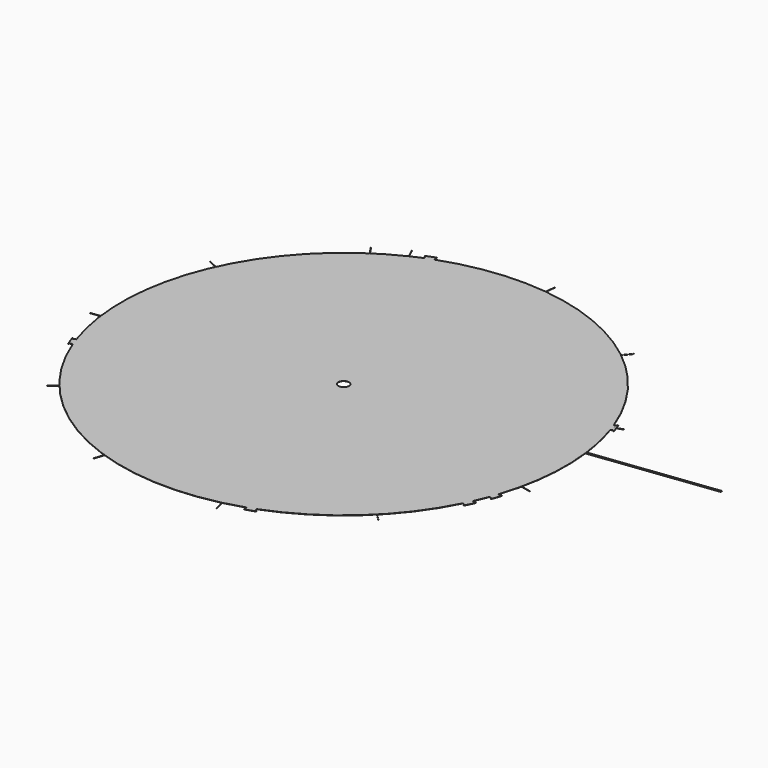
from build123d import *

# Parameters (mm, degrees)
F1_DEPTH = 25.4
F2_R     = 647.7634116636
F3_DEPTH = 25.401
F4_DEPTH = 25.4
F5_COUNT = 12
F5_ANGLE = 352
F6_DEPTH = 25.4


# Not quite as in the source:
# - a feature names something its author has since deleted; it is built from what else it names


with BuildPart() as f1:
    # F0 (on Top) → F1 (new body)
    with BuildSketch(Plane.XY):
        with BuildLine():
            ThreePointArc((26581.7811350736, -5958.878580492), (27076.0679663897, -2997.6433626178), (27241.5, 0))
            ThreePointArc((27241.5, 0), (27192.4503772419, 1634.0026717349), (27045.4781413478, 3262.1211436546))
            Line((27045.4781413478, 3262.1211436546), (27038.1674766005, 3322.1712414177))
            ThreePointArc((27038.1674766005, 3322.1712414177), (27037.0795725779, 3330.3759714052), (27036.1058084748, 3338.5950293075))
            Line((27036.1058084748, 3338.5950293075), (27020.3930406274, 3463.767050483))
            ThreePointArc((27020.3930406274, 3463.767050483), (26566.042215611, 6028.6584949201), (25868.7948916266, 8538.4291942343))
            ThreePointArc((25868.7948916266, 8538.4291942343), (25785.7588811485, 8786.0093997942), (25700.3534370753, 9032.7822656928))
            ThreePointArc((25700.3534370753, 9032.7822656928), (25616.6335659034, 9267.545899548), (25530.7692626016, 9501.5337240783))
            ThreePointArc((25530.7692626016, 9501.5337240783), (22069.8067791267, 15969.4380296244), (17008.4904706443, 21279.3461873245))
            ThreePointArc((17008.4904706443, 21279.3461873245), (10484.2276785736, 25143.1957442532), (3147.6824871739, 27059.0357775354))
            ThreePointArc((3147.6824871739, 27059.0357775354), (-3180.6458046722, 27055.1809181757), (-9337.3289859723, 25591.2799534865))
            ThreePointArc((-9337.3289859723, 25591.2799534865), (-9812.9319890637, 25412.7072156433), (-10285.1222620802, 25225.2964760389))
            ThreePointArc((-10285.1222620802, 25225.2964760389), (-10981.6553363056, 24929.9532355075), (-11669.7181895388, 24615.3813626104))
            Line((-11669.7181895388, 24615.3813626104), (-11694.1794219061, 24603.7698310293))
            ThreePointArc((-11694.1794219061, 24603.7698310293), (-13359.8135246141, 23740.5708616608), (-14962.0879305602, 22764.7808469176))
            ThreePointArc((-14962.0879305602, 22764.7808469176), (-20665.0527895609, 17749.7863495497), (-24761.9849194556, 11355.325847313))
            ThreePointArc((-24761.9849194556, 11355.325847313), (-26932.6996094687, 4090.1117339412), (-27016.7600861348, -3491.9903634219))
            ThreePointArc((-27016.7600861348, -3491.9903634219), (-26537.9717507115, -6151.0468709349), (-25798.1369417149, -8749.5972813909))
            ThreePointArc((-25798.1369417149, -8749.5972813909), (-25630.4432474664, -9229.2849770936), (-25453.8311641421, -9705.7612435783))
            ThreePointArc((-25453.8311641421, -9705.7612435783), (-23563.6007310159, -13669.5297226812), (-21061.0389912676, -17278.0774063061))
            ThreePointArc((-21061.0389912676, -17278.0774063061), (-15482.6864890933, -22413.9630884511), (-8704.7879531066, -25813.2909359006))
            ThreePointArc((-8704.7879531066, -25813.2909359006), (-1252.4719720801, -27212.6925571351), (6296.8812891127, -26503.7470611388))
            ThreePointArc((6296.8812891127, -26503.7470611388), (7526.087542552, -26181.2400117306), (8738.915501307, -25801.7572678881))
            ThreePointArc((8738.915501307, -25801.7572678881), (9218.6681255216, -25634.2637936316), (9695.2130745943, -25457.8507672627))
            ThreePointArc((9695.2130745943, -25457.8507672627), (14879.2922381078, -22818.9829909877), (19384.9043310167, -19139.6135365198))
            ThreePointArc((19384.9043310167, -19139.6135365198), (22160.1999290659, -15843.7641156964), (24381.1200669519, -12151.555724716))
            ThreePointArc((24381.1200669519, -12151.555724716), (24603.4987154748, -11694.7498138109), (24817.3195457392, -11233.8761260159))
            ThreePointArc((24817.3195457392, -11233.8761260159), (25183.6009790471, -10386.797580493), (25520.9793035129, -9527.7981527564))
            ThreePointArc((25520.9793035129, -9527.7981527564), (25693.4049537871, -9052.5280519151), (25856.9806436038, -8574.1398546034))
            ThreePointArc((25856.9806436038, -8574.1398546034), (26251.9681567532, -7275.5405398372), (26581.7811350736, -5958.878580492))
        make_face()
        with BuildLine():
            Line((26219.4698221007, -8697.857158849), (25856.9806436038, -8574.1398546033))
            ThreePointArc((25856.9806436038, -8574.1398546034), (25693.4049537871, -9052.5280519151), (25520.9793035129, -9527.7981527564))
            Line((25520.9793035128, -9527.7981527565), (25892.889499643, -9654.7308437612))
            Line((25892.889499643, -9654.7308437612), (26219.4698221007, -8697.857158849))
        make_face()
        Polygon((26260.4914258481, -8577.6646964148), (26219.4698221007, -8697.857158849), (25892.889499643, -9654.7308437612), (25850.2700590491, -9779.6049355713), (25922.390865835, -9804.2022830051), (26127.4988845718, -9203.2399708342), (26332.6069033086, -8602.2776586632), align=None)
        with BuildLine():
            Line((25167.4813878364, -11405.5197307459), (24817.3195457391, -11233.876126016))
            ThreePointArc((24817.3195457392, -11233.8761260159), (24603.4987154748, -11694.7498138109), (24381.1200669519, -12151.555724716))
            Line((24381.1200669517, -12151.5557247163), (24720.2908078015, -12317.8116714798))
            Line((24720.2908078015, -12317.8116714798), (25167.4813878364, -11405.5197307459))
        make_face()
        with BuildLine():
            ThreePointArc((25700.3534370753, 9032.7822656928), (25785.7588811485, 8786.0093997942), (25868.7948916266, 8538.4291942343))
            Line((25868.7948916267, 8538.4291942341), (26198.5379395342, 8651.0553115066))
            Line((26198.5379395342, 8651.0553115066), (26028.7355470907, 9148.1971803935))
            Line((26028.7355470907, 9148.1971803935), (25700.3534370753, 9032.7822656928))
        make_face()
        Polygon((25223.3802103407, -11291.4832381542), (25167.4813878364, -11405.5197307459), (24720.2908078015, -12317.8116714798), (24664.3847231965, -12431.8629791328), (24732.8138808522, -12465.3874575742), (25012.307993374, -11895.2049946155), (25291.8021058958, -11325.0225316568), align=None)
        with BuildLine():
            ThreePointArc((25530.7692626016, 9501.5337240783), (25616.6335659034, 9267.545899548), (25700.3534370753, 9032.7822656928))
            Line((25700.3534370753, 9032.7822656928), (26028.7355470907, 9148.1971803935))
            Line((26028.7355470907, 9148.1971803935), (25868.6350307326, 9616.9342150529))
            Line((25868.6350307326, 9616.9342150529), (25530.7692626015, 9501.5337240786))
        make_face()
        Polygon((26028.7355470907, 9148.1971803935), (26198.5379395342, 8651.0553115066), (26238.0846514917, 8535.2717468115), (26310.1891088702, 8559.9169795832), (26104.9422822996, 9160.8318988377), (26100.62746037, 9173.4646927998), align=None)
        Polygon((25868.6350307326, 9616.9342150529), (26028.7355470907, 9148.1971803935), (26100.62746037, 9173.4646927998), (25899.695455729, 9761.7468180923), (25827.5856654185, 9737.1171989038), align=None)
        with BuildLine():
            Line((9817.5292529223, -25823.5618318769), (9695.2130745944, -25457.8507672626))
            ThreePointArc((9695.2130745943, -25457.8507672627), (9218.6681255216, -25634.2637936316), (8738.915501307, -25801.7572678881))
            Line((8738.9155013075, -25801.7572678879), (8853.993553604, -26145.8271823865))
            Line((8853.993553604, -26145.8271823865), (9817.5292529223, -25823.5618318769))
        make_face()
        Polygon((9937.9712153371, -25783.2786630632), (9817.5292529223, -25823.5618318769), (8853.993553604, -26145.8271823865), (8733.5359439607, -26186.1155845918), (8757.7214924774, -26258.3755286491), (9359.9313045514, -26056.9596845806), (9962.1411166253, -25855.5438405121), align=None)
        with BuildLine():
            ThreePointArc((-10285.1222620802, 25225.2964760389), (-9812.9319890637, 25412.7072156433), (-9337.3289859723, 25591.2799534865))
            Line((-9337.3289859723, 25591.2799534865), (-9480.2259121424, 25961.3424129862))
            Line((-9480.2259121424, 25961.3424129862), (-10428.0191882503, 25595.3589355386))
            Line((-10428.0191882503, 25595.3589355386), (-10285.1222620802, 25225.2964760389))
        make_face()
        Polygon((-10428.0191882503, 25595.3589355386), (-9480.2259121424, 25961.3424129862), (-9361.7363610477, 26007.0962910142), (-9389.2005134374, 26078.1748433752), (-9981.5713110049, 25849.4351699704), (-10573.9421085723, 25620.6954965657), (-10546.4933477638, 25549.6110008576), align=None)
        with BuildLine():
            Line((-25797.5388182234, -9838.4814533939), (-25453.8311641418, -9705.7612435791))
            ThreePointArc((-25453.8311641421, -9705.7612435783), (-25630.4432474664, -9229.2849770936), (-25798.1369417149, -8749.5972813909))
            Line((-25798.1369417149, -8749.5972813911), (-26163.522295671, -8890.688177286))
            Line((-26163.522295671, -8890.688177286), (-25797.5388182234, -9838.4814533939))
        make_face()
        Polygon((-25751.7908835424, -9956.9556129074), (-25797.5388182234, -9838.4814533939), (-26163.522295671, -8890.688177286), (-26209.276173699, -8772.1986261914), (-26280.35472606, -8799.6627785811), (-26051.6150526553, -9392.0335761485), (-25822.8753792505, -9984.404373716), align=None)
    extrude(amount=F1_DEPTH)

    # F2 (on face) → F3 (cut, through all)
    with BuildSketch(Plane.XY.offset(25.4)):
        Circle(F2_R)
    extrude(amount=-F3_DEPTH, mode=Mode.SUBTRACT)


with BuildPart() as f1b:
    # F0 (on Top) → F1, piece 2 (new body)
    with BuildSketch(Plane.XY):
        with BuildLine():
            ThreePointArc((27038.1674766005, 3322.1712414177), (27041.8394776597, 3292.1482218279), (27045.4781413478, 3262.1211436546))
            Line((27045.4781413478, 3262.1211436546), (36395.7287217049, 4410.9835288363))
            Line((36395.7287217049, 4410.9835288363), (36388.3513912897, 4471.0254354095))
            Line((36388.3513912896, 4471.0254354095), (27038.1674766005, 3322.1712414177))
        make_face()
        with BuildLine():
            ThreePointArc((27035.8130126605, 3341.2777487745), (27036.9919324044, 3331.7247030777), (27038.1674766005, 3322.1712414177))
            Line((27038.1674766005, 3322.1712414177), (36388.3513912896, 4471.0254354095))
            Line((36388.3513912897, 4471.0254354095), (36370.9479572001, 4612.6668293611))
            Line((36370.9479572001, 4612.6668293611), (27020.3930406274, 3463.767050483))
            ThreePointArc((27020.3930406274, 3463.767050483), (27028.1724155767, 3402.5311348847), (27035.8130126605, 3341.2777487745))
        make_face()
    extrude(amount=F1_DEPTH)

    # F0 (on Top) → F6 (join)
    with BuildSketch(Plane.XY):
        with BuildLine():
            ThreePointArc((27035.8130126605, 3341.2777487745), (27036.9919324044, 3331.7247030777), (27038.1674766005, 3322.1712414177))
            Line((27038.1674766005, 3322.1712414177), (36388.3513912896, 4471.0254354095))
            Line((36388.3513912897, 4471.0254354095), (36370.9479572001, 4612.6668293611))
            Line((36370.9479572001, 4612.6668293611), (27020.3930406274, 3463.767050483))
            ThreePointArc((27020.3930406274, 3463.767050483), (27028.1724155767, 3402.5311348847), (27035.8130126605, 3341.2777487745))
        make_face()
        Polygon((36388.3513912897, 4471.0254354095), (36395.7287217049, 4410.9835288363), (42171.4213444891, 5120.6410878143), (42146.6405799844, 5322.3243883391), (36370.9479572001, 4612.6668293611), align=None)
    extrude(amount=F6_DEPTH)


with BuildPart() as f4:
    # F0 (on Top) → F4 (new body)
    with BuildSketch(Plane.XY):
        with BuildLine():
            ThreePointArc((-11694.1794219061, 24603.7698310293), (-11681.9502484147, 24609.5786360426), (-11669.7181895388, 24615.3813626104))
            Line((-11669.7181895388, 24615.3813626104), (-12213.7609955779, 25762.9515893055))
            Line((-12213.7609955779, 25762.9515893055), (-12237.8474886915, 25750.5496059335))
            Line((-12237.8474886915, 25750.5496059335), (-11694.1794219061, 24603.7698310293))
        make_face()
    extrude(amount=F4_DEPTH)


with BuildPart() as f5_1:
    # F5: instance of F4
    add(f4.part.rotate(Axis((0, 0, 0), (0, 0, -1)), 1 * F5_ANGLE / (F5_COUNT - 1)))


with BuildPart() as f5_2:
    # F5: instance of F4
    add(f4.part.rotate(Axis((0, 0, 0), (0, 0, -1)), 2 * F5_ANGLE / (F5_COUNT - 1)))


with BuildPart() as f5_3:
    # F5: instance of F4
    add(f4.part.rotate(Axis((0, 0, 0), (0, 0, -1)), 3 * F5_ANGLE / (F5_COUNT - 1)))


with BuildPart() as f5_4:
    # F5: instance of F4
    add(f4.part.rotate(Axis((0, 0, 0), (0, 0, -1)), 4 * F5_ANGLE / (F5_COUNT - 1)))


with BuildPart() as f5_5:
    # F5: instance of F4
    add(f4.part.rotate(Axis((0, 0, 0), (0, 0, -1)), 5 * F5_ANGLE / (F5_COUNT - 1)))


with BuildPart() as f5_6:
    # F5: instance of F4
    add(f4.part.rotate(Axis((0, 0, 0), (0, 0, -1)), 6 * F5_ANGLE / (F5_COUNT - 1)))


with BuildPart() as f5_7:
    # F5: instance of F4
    add(f4.part.rotate(Axis((0, 0, 0), (0, 0, -1)), 7 * F5_ANGLE / (F5_COUNT - 1)))


with BuildPart() as f5_8:
    # F5: instance of F4
    add(f4.part.rotate(Axis((0, 0, 0), (0, 0, -1)), 8 * F5_ANGLE / (F5_COUNT - 1)))


with BuildPart() as f5_9:
    # F5: instance of F4
    add(f4.part.rotate(Axis((0, 0, 0), (0, 0, -1)), 9 * F5_ANGLE / (F5_COUNT - 1)))


with BuildPart() as f5_10:
    # F5: instance of F4
    add(f4.part.rotate(Axis((0, 0, 0), (0, 0, -1)), 10 * F5_ANGLE / (F5_COUNT - 1)))


with BuildPart() as f5_11:
    # F5: instance of F4
    add(f4.part.rotate(Axis((0, 0, 0), (0, 0, -1)), 11 * F5_ANGLE / (F5_COUNT - 1)))


solid = Compound([f1.part, f1b.part, f4.part, f5_1.part, f5_2.part, f5_3.part, f5_4.part, f5_5.part, f5_6.part, f5_7.part, f5_8.part, f5_9.part, f5_10.part, f5_11.part])
